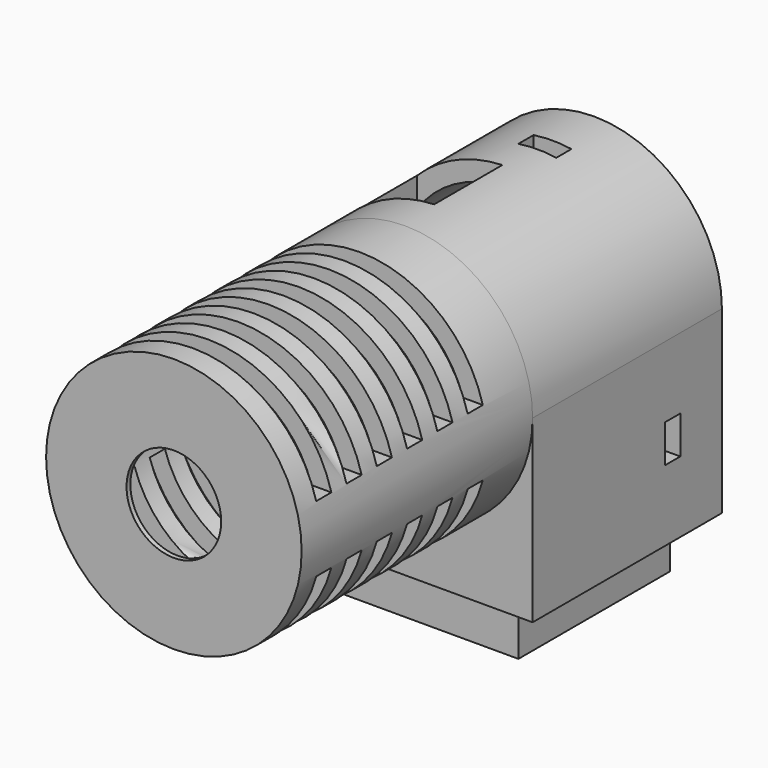
from build123d import *
from build123d import SkipClean  # not in build123d's __all__

# Parameters (mm, degrees)
F0_R      = 13.5
F0_R_2    = 11.5
F1_DEPTH  = 30
F2_R      = 13.5
F2_R_2    = 5
F3_DEPTH  = 0.5
F5_W      = 27
F5_H      = 2
F6_DEPTH  = 10
F8_W      = 27
F8_H      = 2
F9_DEPTH  = 10
F11_DEPTH = 25
F13_DEPTH = 1
F14_W     = 20
F14_H     = 20
F15_DEPTH = 5.55625
F16_W     = 4
F16_H     = 2
F17_DEPTH = 3
F18_W     = 2
F18_H     = 4
F19_DEPTH = 2
F20_W     = 2
F20_H     = 4
F21_DEPTH = 2
F22_W     = 9
F22_H     = 9
F23_DEPTH = 8


# Not quite as in the source:
# - after a boolean that leaves OpenCascade's solid faulty, fix() repairs it
# - a length typed as a fraction of an inch, garbled in the dataset ("3 / 203.2 mm" for 3/8 in), is restored


with BuildPart() as f1:
    # F0 (on Front) → F1 (new body)
    with BuildSketch(Plane.XZ):
        Circle(F0_R)
        Circle(F0_R_2, mode=Mode.SUBTRACT)
    extrude(amount=-F1_DEPTH)

    # F2 (on Front) → F3 (join)
    with BuildSketch(Plane.XZ):
        Circle(F2_R)
        Circle(F2_R_2, mode=Mode.SUBTRACT)
    extrude(amount=F3_DEPTH)

    # F5 (on offset) → F6 (cut)
    with BuildSketch(Plane.XY.offset(13.5)):
        with Locations((0, 2.9999998671)):
            Rectangle(F5_W, F5_H)
        with Locations((0, 22.9999998671)):
            Rectangle(F5_W, F5_H)
        with Locations((0, 6.9999998671)):
            Rectangle(F5_W, F5_H)
        with Locations((0, 10.9999998671)):
            Rectangle(F5_W, F5_H)
        with Locations((0, 14.9999998671)):
            Rectangle(F5_W, F5_H)
        with Locations((0, 18.9999998671)):
            Rectangle(F5_W, F5_H)
    extrude(amount=-F6_DEPTH, mode=Mode.SUBTRACT)

    # F8 (on offset) → F9 (cut)
    with BuildSketch(Plane.XY.offset(-13.5)):
        with Locations((5.811e-07, 3.000000095)):
            Rectangle(F8_W, F8_H)
        with Locations((5.811e-07, 7.000000095)):
            Rectangle(F8_W, F8_H)
        with Locations((5.811e-07, 11.000000095)):
            Rectangle(F8_W, F8_H)
        with Locations((5.811e-07, 15.000000095)):
            Rectangle(F8_W, F8_H)
        with Locations((5.811e-07, 19.000000095)):
            Rectangle(F8_W, F8_H)
        with Locations((5.811e-07, 23.000000095)):
            Rectangle(F8_W, F8_H)
    extrude(amount=F9_DEPTH, mode=Mode.SUBTRACT)

    # F10 (on face) → F11 (join)
    with BuildSketch(Plane(origin=(0, 30, 0), x_dir=(-1, 0, 0), z_dir=(0, 1, 0))):
        with BuildLine():
            Line((11.5, 0), (11.5, -7.0710678119))
            ThreePointArc((11.5, -7.0710678119), (12.9903810568, -3.6742346142), (13.5, 0))
            ThreePointArc((13.5, 0), (0, 13.5), (-13.5, 0))
            ThreePointArc((-13.5, 0), (-12.9903810568, -3.6742346142), (-11.5, -7.0710678119))
            Line((-11.5, -7.0710678119), (-11.5, 0))
            ThreePointArc((-11.5, 0), (0, 11.5), (11.5, 0))
        make_face()
        with BuildLine():
            ThreePointArc((13.5, 0), (12.9903810568, -3.6742346142), (11.5, -7.0710678119))
            Line((11.5, -7.0710678119), (11.5, -17))
            Line((11.5, -17), (-11.5, -17))
            Line((-11.5, -17), (-11.5, -7.0710678119))
            ThreePointArc((-11.5, -7.0710678119), (-12.9903810568, -3.6742346142), (-13.5, 0))
            Line((-13.5, 0), (-13.5, -19))
            Line((-13.5, -19), (13.5, -19))
            Line((13.5, -19), (13.5, 0))
        make_face()
    with SkipClean():  # cleaning this boolean's faces spoils the solid; the shape is the same uncleaned
        extrude(amount=F11_DEPTH)

    # F12 (on face) → F13 (join)
    with BuildSketch(Plane(origin=(0, 30, 0), x_dir=(-1, 0, 0), z_dir=(0, 1, 0))):
        with BuildLine():
            Line((13.5, -19), (13.5, 0))
            ThreePointArc((13.5, 0), (12.9903810568, -3.6742346142), (11.5, -7.0710678119))
            ThreePointArc((11.5, -7.0710678119), (0, -13.5), (-11.5, -7.0710678119))
            ThreePointArc((-11.5, -7.0710678119), (-12.9903810568, -3.6742346142), (-13.5, 0))
            Line((-13.5, 0), (-13.5, -19))
            Line((-13.5, -19), (13.5, -19))
        make_face()
        with BuildLine():
            ThreePointArc((-11.5, -7.0710678119), (0, -13.5), (11.5, -7.0710678119))
            Line((11.5, -7.0710678119), (11.5, 0))
            ThreePointArc((11.5, 0), (0, -11.5), (-11.5, 0))
            Line((-11.5, 0), (-11.5, -7.0710678119))
        make_face()
    with SkipClean():  # cleaning this boolean's faces spoils the solid; the shape is the same uncleaned
        extrude(amount=F13_DEPTH)

    # F14 (on face) → F15 (join)
    with BuildSketch(Plane(origin=(0, 0, -19), x_dir=(1, 0, 0), z_dir=(0, 0, -1))):
        with Locations((0, -42.5)):
            Rectangle(F14_W, F14_H)
        Polygon((-3.6661742094, -36.15), (3.6661742094, -36.15), (7.3323484187, -42.5), (3.6661742094, -48.85), (-3.6661742094, -48.85), (-7.3323484187, -42.5), align=None, mode=Mode.SUBTRACT)
    extrude(amount=F15_DEPTH)

    add(f1.part.fix(), mode=Mode.REPLACE)

    # F16 (on offset) → F17 (cut)
    with BuildSketch(Plane.XY.offset(13.5)):
        with Locations((0, 48.5)):
            Rectangle(F16_W, F16_H)
    extrude(amount=-F17_DEPTH, mode=Mode.SUBTRACT)

    # F18 (on face) → F19 (cut)
    with BuildSketch(Plane.YZ.offset(13.5)):
        with Locations((48.5, -9.5)):
            Rectangle(F18_W, F18_H)
    extrude(amount=-F19_DEPTH, mode=Mode.SUBTRACT)

    # F20 (on face) → F21 (cut)
    with BuildSketch(Plane(origin=(-13.5, 0, 0), x_dir=(0, -1, 0), z_dir=(-1, 0, 0))):
        with Locations((-48.5, -9.5)):
            Rectangle(F20_W, F20_H)
    extrude(amount=-F21_DEPTH, mode=Mode.SUBTRACT)

    # F22 (on offset) → F23 (cut)
    with BuildSketch(Plane.XY.offset(13.5)):
        with Locations((-5, 39)):
            Rectangle(F22_W, F22_H)
    extrude(amount=-F23_DEPTH, mode=Mode.SUBTRACT)


solid = f1.part
